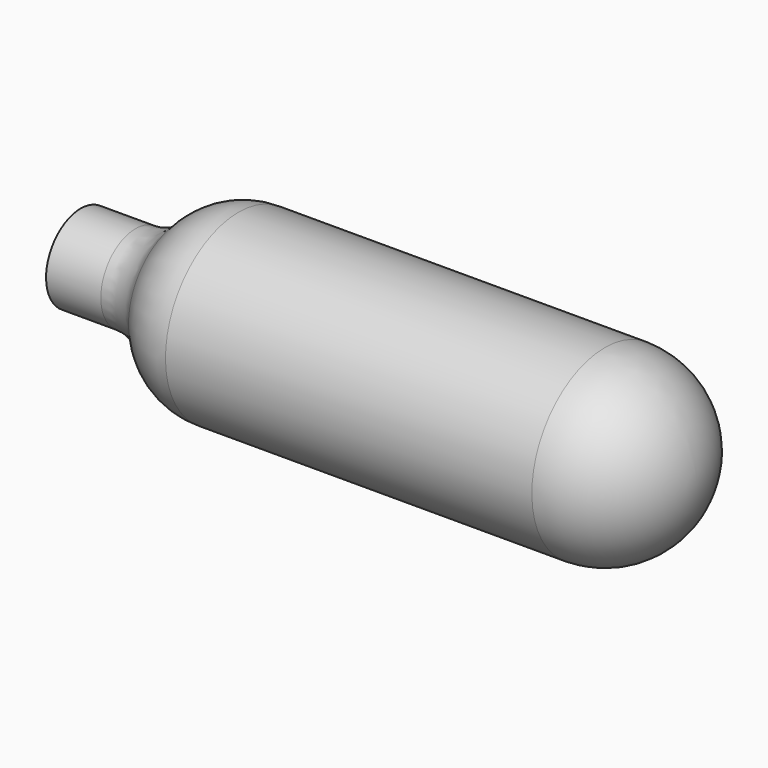
from build123d import *

# Parameters (mm, degrees)
F3_R = 6
F4_R = 9.5


# Not quite as in the source:
# - a fillet or chamfer that OpenCascade refuses, or shapes differently, is made with other operations: its cross-section is extruded or revolved along the edge and cut away or added


with BuildPart() as f1:
    # F0 (on Front) → F1 (revolve)
    with BuildSketch(Plane.XZ):
        Polygon((0, 4.5), (0, 0), (64, 0), (64, 9.5), (9, 9.5), (9, 4.5), align=None)
    revolve(axis=Axis((32, 0, 0), (1, 0, 0)))

    # F2: fillet of radius 8 on 1 edges, made by hand

    # F2_s1 → F2_t2 (revolve, cut)
    with BuildSketch(Plane.XZ):
        with BuildLine():
            ThreePointArc((16.4161984871, 9.5), (11.9440625321, 8.1332495807), (9, 4.5))
            Line((9, 4.5), (9, 9.5))
            Line((9, 9.5), (16.4161984871, 9.5))
        make_face()
    revolve(axis=Axis((9, 0, 0), (1, 0, 0)), mode=Mode.SUBTRACT)

    # F3
    f3_edges = [f1.edges().sort_by_distance(p)[0] for p in [
        (9, 0, -4.5),
    ]]
    fillet(f3_edges, radius=F3_R)

    # F4
    f4_edges = [f1.edges().sort_by_distance(p)[0] for p in [
        (64, 0, -9.5),
    ]]
    fillet(f4_edges, radius=F4_R)


solid = f1.part
